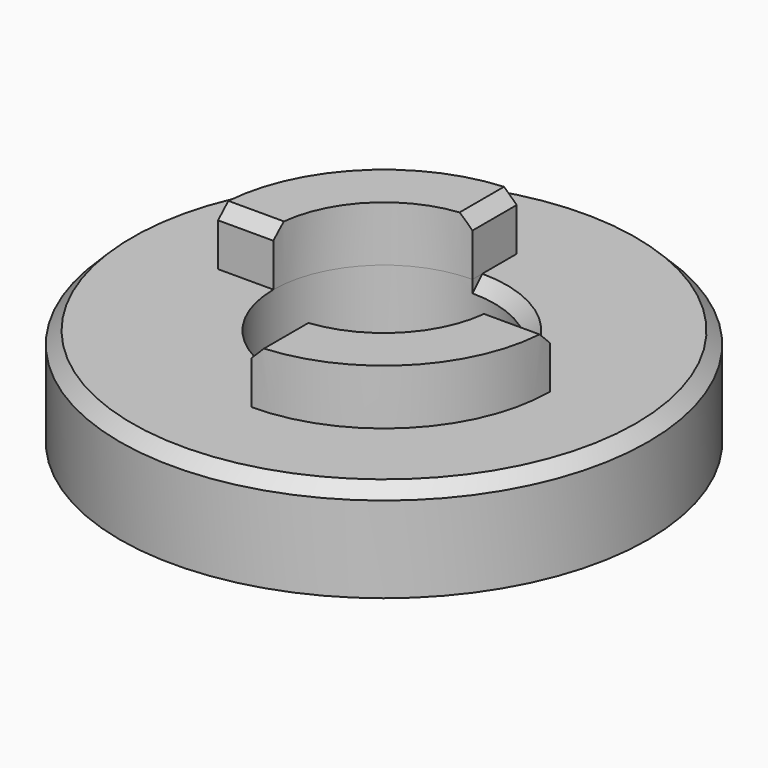
from build123d import *

# Parameters (mm, degrees)
F0_R         = 10.75
F0_R_2       = 4.5
F1_DEPTH     = 4
F2_R         = 6.75
F2_R_2       = 4.5
F3_DEPTH     = 6.25
F4_W         = 12
F4_H         = 12
F5_DEPTH     = 10
F8_T1_DEPTH  = 4.821682988
F8_T3_DEPTH  = 4.821682988
F8_T5_DEPTH  = 4.821682988
F8_T7_DEPTH  = 4.821682988
F8_T12_ANGLE = 90


# Not quite as in the source:
# - a fillet or chamfer that OpenCascade refuses, or shapes differently, is made with other operations: its cross-section is extruded or revolved along the edge and cut away or added


with BuildPart() as f1:
    # F0 (on Top) → F1 (new body)
    with BuildSketch(Plane.XY):
        Circle(F0_R)
        Circle(F0_R_2, mode=Mode.SUBTRACT)
    extrude(amount=F1_DEPTH)


with BuildPart() as f3:
    # F2 (on Top) → F3 (new body)
    with BuildSketch(Plane.XY):
        Circle(F2_R)
        Circle(F2_R_2, mode=Mode.SUBTRACT)
    extrude(amount=F3_DEPTH)


with BuildPart() as f5:
    # F4 (on Top) → F5 (new body)
    with BuildSketch(Plane.XY):
        with Locations((6, 6)):
            Rectangle(F4_W, F4_H)
    extrude(amount=F5_DEPTH)


with BuildPart() as f5b:
    # F4 (on Top) → F5, piece 2 (new body)
    with BuildSketch(Plane.XY):
        with Locations((-6, -6)):
            Rectangle(F4_W, F4_H)
    extrude(amount=F5_DEPTH)


with BuildPart() as f3_1:
    add(f3.part)

    # F6: cut F5b, F5
    add(f5b.part, mode=Mode.SUBTRACT)
    add(f5.part, mode=Mode.SUBTRACT)


with BuildPart() as f1_1:
    add(f1.part)

    # F7: union F3
    add(f3_1.part)

    # F8: chamfer of 0.5 on 6 edges, made by hand

    # F8_s2 → F8_t1 (cut)
    with BuildSketch(Plane.YZ.offset(-8.035841494)):
        Polygon((0, 5.75), (0.5, 6.25), (0, 6.25), align=None)
    extrude(amount=F8_T1_DEPTH, mode=Mode.SUBTRACT)

    # F8_s4 → F8_t3 (cut)
    with BuildSketch(Plane.XZ.offset(-8.035841494)):
        Polygon((-0.5, 6.25), (0, 5.75), (0, 6.25), align=None)
    extrude(amount=F8_T3_DEPTH, mode=Mode.SUBTRACT)

    # F8_s6 → F8_t5 (cut)
    with BuildSketch(Plane.XZ.offset(3.214158506)):
        Polygon((0.5, 6.25), (0, 5.75), (0, 6.25), align=None)
    extrude(amount=F8_T5_DEPTH, mode=Mode.SUBTRACT)

    # F8_s8 → F8_t7 (cut)
    with BuildSketch(Plane.YZ.offset(3.214158506)):
        Polygon((0, 5.75), (-0.5, 6.25), (0, 6.25), align=None)
    extrude(amount=F8_T7_DEPTH, mode=Mode.SUBTRACT)

    # F8_s9 → F8_t10 (revolve, cut)
    with BuildSketch(Plane.XZ):
        Polygon((10.75, 3.5), (10.25, 4), (10.75, 4), align=None)
    revolve(axis=Axis((0, 0, 4), (0, 0, 1)), mode=Mode.SUBTRACT)

    # F8_s11 → F8_t12 (revolve, cut)
    with BuildSketch(Plane.XZ):
        Polygon((5, 4), (4.5, 3.5), (4.5, 4), align=None)
    revolve(axis=Axis((0, 0, 4), (0, 0, 1)), revolution_arc=F8_T12_ANGLE, mode=Mode.SUBTRACT)


solid = f1_1.part
